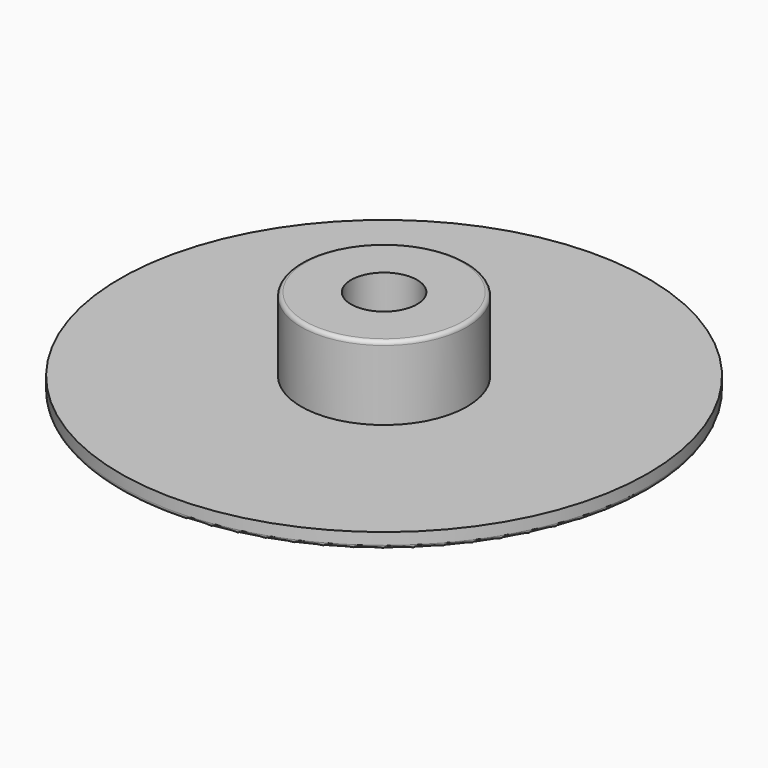
from build123d import *

# Parameters (mm, degrees)
F0_R     = 20.37
F0_R_2   = 6.4
F0_R_3   = 2.55
F1_DEPTH = 1.2
F2_DEPTH = 5.7
F3_R     = 0.3


# Not quite as in the source:
# - a feature names something its author has since deleted; it is built from what else it names


with BuildPart() as f1:
    # F0 (on Top) → F1 (new body)
    with BuildSketch(Plane.XY):
        Circle(F0_R)
        Circle(F0_R_2, mode=Mode.SUBTRACT)
        Circle(F0_R_2)
        Circle(F0_R_3, mode=Mode.SUBTRACT)
    extrude(amount=-F1_DEPTH)

    # F0 (on Top) → F2 (join)
    with BuildSketch(Plane.XY):
        Circle(F0_R_2)
        Circle(F0_R_3, mode=Mode.SUBTRACT)
    extrude(amount=F2_DEPTH)

    # F3
    f3_edges = [f1.edges().sort_by_distance(p)[0] for p in [
        (-20.37, 0, -1.2),
        (-6.4, 0, 5.7),
    ]]
    fillet(f3_edges, radius=F3_R)


solid = f1.part
